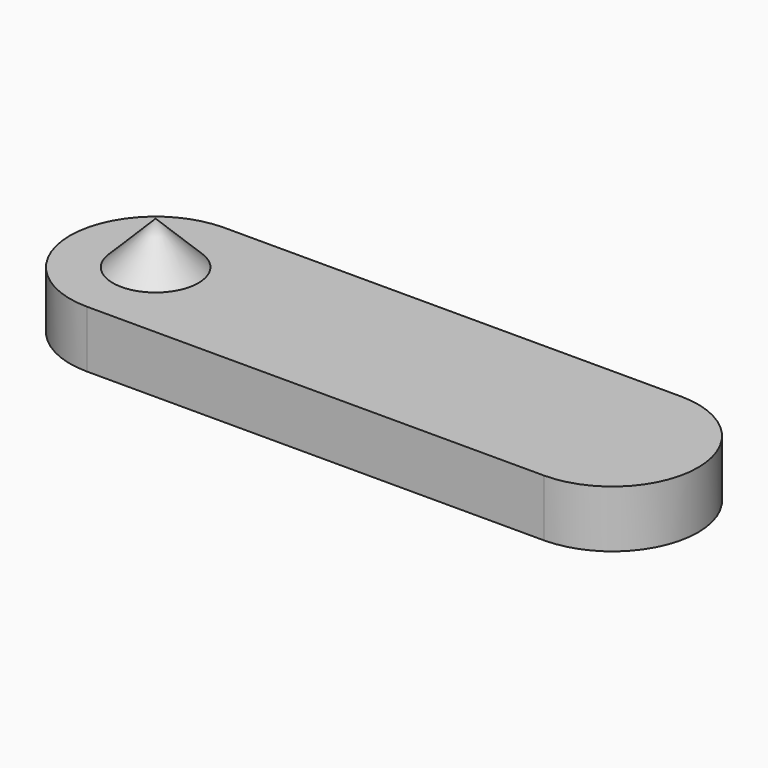
from build123d import *

# Parameters (mm, degrees)
F1_DEPTH = 10
F2_R     = 7.5
F3_DEPTH = 7.5
F3_TAPER = 45
F4_R     = 7.5


# Not quite as in the source:
# - an extrude whose draft closes it to a point is written as a loft to that point


with BuildPart() as f1:
    # F0 (on Top) → F1 (new body)
    with BuildSketch(Plane.XY):
        with BuildLine():
            Line((51.71875, 3.3977172854), (-28.28125, 3.3977172854))
            ThreePointArc((-28.28125, 3.3977172854), (-43.28125, -11.6022827146), (-28.28125, -26.6022827146))
            Line((-28.28125, -26.6022827146), (51.71875, -26.6022827146))
            ThreePointArc((51.71875, -26.6022827146), (66.71875, -11.6022827146), (51.71875, 3.3977172854))
        make_face()
    extrude(amount=F1_DEPTH)

    # F2 (on face) → F3 (join)
    with BuildSketch(Plane.XY.offset(10)):
        with Locations((-28.28125, -11.6022827146)):
            Circle(F2_R)
    extrude(amount=F3_DEPTH, taper=F3_TAPER)

    # F4 (on face) → F5 section 0
    with BuildSketch(Plane(origin=(0, 0, 0), x_dir=(1, 0, 0), z_dir=(0, 0, -1)), mode=Mode.PRIVATE) as f5_s0:
        with Locations((51.71875, 11.6022827146)):
            Circle(F4_R)
    loft([f5_s0.sketch, Vertex(51.71875, -11.6022827146, 7.5)], ruled=True, mode=Mode.SUBTRACT)


solid = f1.part
